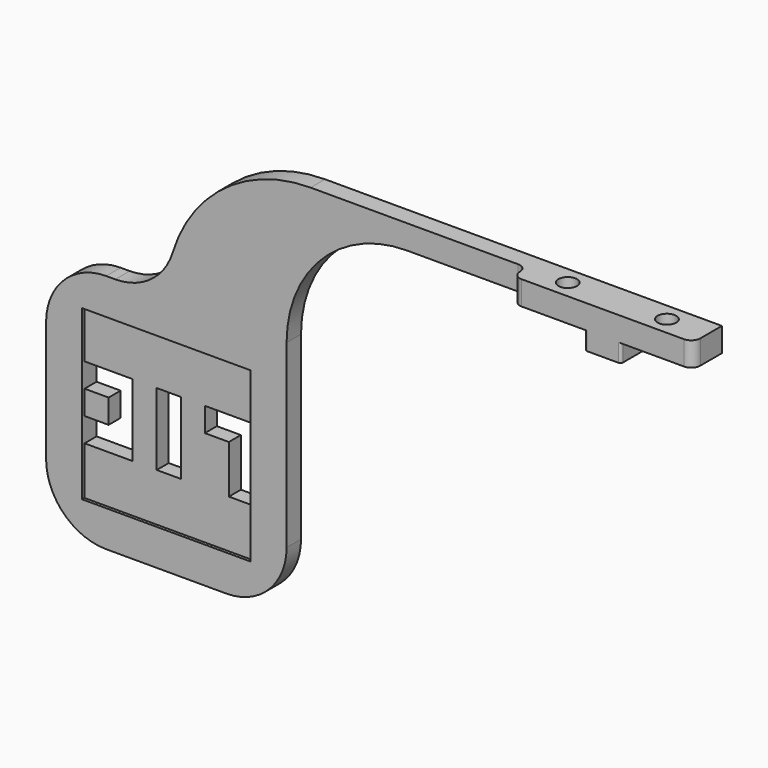
from build123d import *

# Parameters (mm, degrees)
F0_W      = 30
F0_H      = 6
F1_DEPTH  = 4
F2_W      = 6
F2_H      = 6
F3_DEPTH  = 3
F4_R      = 1.55
F5_DEPTH  = 4
F7_DEPTH  = 3
F8_W      = 28
F8_H      = 28
F9_DEPTH  = 0.5
F11_R     = 1.49999
F12_R     = 10
F13_R     = 0.4
F10_W     = 4
F10_H     = 12
F14_DEPTH = 2.5


# Not quite as in the source:
# - a fillet or chamfer is up to 0.001 mm smaller than in the source, because OpenCascade refuses the exact size


with BuildPart() as f1:
    # F0 (on Top) → F1 (new body)
    with BuildSketch(Plane.XY):
        Rectangle(F0_W, F0_H)
    extrude(amount=F1_DEPTH)

    # F2 (on face) → F3 (join)
    with BuildSketch(Plane(origin=(0, 0, 0), x_dir=(1, 0, 0), z_dir=(0, 0, -1))):
        Rectangle(F2_W, F2_H)
    extrude(amount=F3_DEPTH)

    # F4 (on face) → F5 (cut, through all)
    with BuildSketch(Plane.XY.offset(4)):
        with Locations((-8.25, 0)):
            Circle(F4_R)
        with Locations((8.25, 0)):
            Circle(F4_R)
    extrude(amount=-F5_DEPTH, mode=Mode.SUBTRACT)

    # F6 (on Front) → F7 (join, through all)
    with BuildSketch(Plane.XZ):
        with BuildLine():
            Line((-15, 0), (-15, 4))
            Line((-15, 4), (-51, 4))
            ThreePointArc((-51, 4), (-67.9705627485, -3.0294372515), (-75, -20))
            Line((-75, -20), (-95, -20))
            Line((-95, -20), (-95, -60))
            Line((-95, -60), (-55, -60))
            Line((-55, -60), (-55, -20))
            ThreePointArc((-55, -20), (-49.1421356237, -5.8578643763), (-35, 0))
            Line((-35, 0), (-15, 0))
        make_face()
    extrude(amount=-F7_DEPTH)

    # F8 (on face) → F9 (cut)
    with BuildSketch(Plane.XZ):
        with Locations((-75, -40)):
            Rectangle(F8_W, F8_H)
    extrude(amount=-F9_DEPTH, mode=Mode.SUBTRACT)

    # F11 (radius 1.5 in the source; OpenCascade refuses exactly that, so slightly less here)
    f11_edges = [f1.edges().sort_by_distance(p)[0] for p in [
        (-15, 0, 2),
        (-15, -3, 2),
        (15, -3, 2),
    ]]
    fillet(f11_edges, radius=F11_R)

    # F12
    f12_edges = [f1.edges().sort_by_distance(p)[0] for p in [
        (-55, 1.5, -60),
        (-95, 1.5, -60),
        (-95, 1.5, -20),
        (-75, 1.5, -20),
    ]]
    fillet(f12_edges, radius=F12_R)

    # F13
    f13_edges = [f1.edges().sort_by_distance(p)[0] for p in [
        (3, -3, -1.5),
        (3, 3, -1.5),
        (-3, 3, -1.5),
        (-3, -3, -1.5),
    ]]
    fillet(f13_edges, radius=F13_R)

    # F10 (on face) → F14 (cut, through all)
    with BuildSketch(Plane.XZ.offset(-0.5)):
        Polygon((-81, -34), (-89, -34), (-89, -38), (-85, -38), (-85, -42), (-89, -42), (-89, -46), (-81, -46), align=None)
        with Locations((-75, -40)):
            Rectangle(F10_W, F10_H)
        Polygon((-61, -46), (-61, -34), (-69, -34), (-69, -38), (-65, -38), (-65, -46), align=None)
    extrude(amount=-F14_DEPTH, mode=Mode.SUBTRACT)


solid = f1.part
